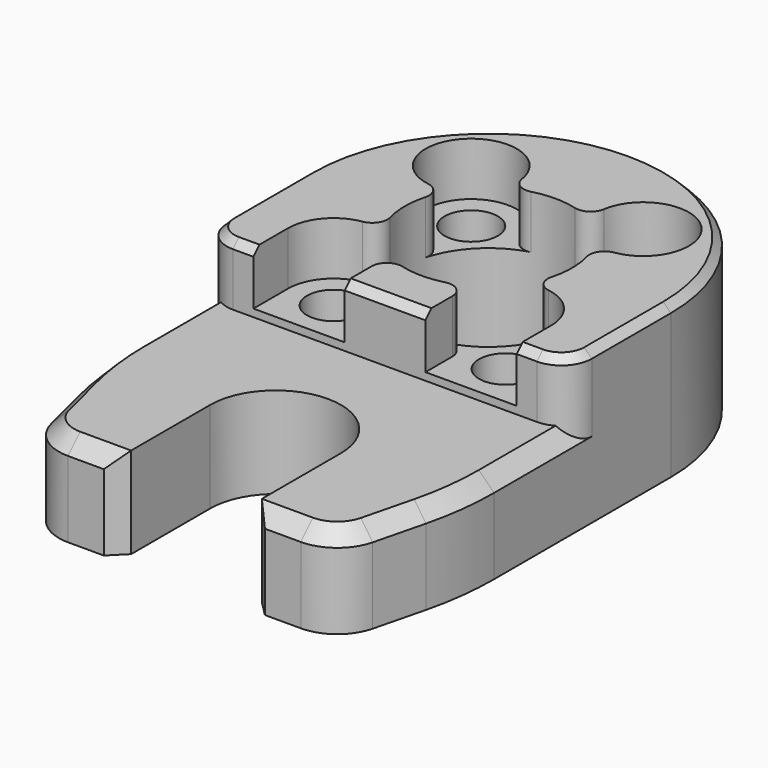
from build123d import *

# Parameters (mm, degrees)
F0_R        = 1.75
F0_R_2      = 5.5
F1_DEPTH    = 10
F2_SIZE2    = 8
F2_SIZE     = 2
F3_SIZE2    = 2
F3_SIZE     = 8
F5_W        = 20
F5_H        = 8
F6_DEPTH    = 15
F7_R        = 3
F8_DEPTH    = 3.5
F9_T1_DEPTH = 7.3998501729
F9_T3_DEPTH = 7.1931423334
F10_R       = 2
F11_SIZE    = 0.5
F12_SIZE    = 1
F13_R       = 3
F14_R       = 20
F15_SIZE    = 1
F17_ANGLE   = 45


# Not quite as in the source:
# - a fillet or chamfer that OpenCascade refuses, or shapes differently, is made with other operations: its cross-section is extruded or revolved along the edge and cut away or added


with BuildPart() as f1:
    # F0 (on Top) → F1 (new body)
    with BuildSketch(Plane.XY):
        with BuildLine():
            Line((-9.1923881554, -26.1629509039), (8.4852813742, -8.4852813742))
            ThreePointArc((8.4852813742, -8.4852813742), (8.4852813742, 8.4852813742), (-8.4852813742, 8.4852813742))
            Line((-8.4852813742, 8.4852813742), (-26.1629509039, -9.1923881554))
            Line((-26.1629509039, -9.1923881554), (-20.7182286888, -14.6371103706))
            Line((-20.7182286888, -14.6371103706), (-15.4149278299, -9.3338095117))
            ThreePointArc((-15.4149278299, -9.3338095117), (-9.3338095117, -9.3338095117), (-9.3338095117, -15.4149278299))
            Line((-9.3338095117, -15.4149278299), (-14.6371103706, -20.7182286888))
            Line((-14.6371103706, -20.7182286888), (-9.1923881554, -26.1629509039))
        make_face()
        with Locations((0, -8)):
            Circle(F0_R, mode=Mode.SUBTRACT)
        with Locations((-8, 0)):
            Circle(F0_R, mode=Mode.SUBTRACT)
        Circle(F0_R_2, mode=Mode.SUBTRACT)
        with Locations((8, 0)):
            Circle(F0_R, mode=Mode.SUBTRACT)
        with Locations((0, 8)):
            Circle(F0_R, mode=Mode.SUBTRACT)
    extrude(amount=F1_DEPTH)

    # F2
    f2_edges = [f1.edges().sort_by_distance(p)[0] for p in [
        (-26.162951, -9.192388, 5),
    ]]
    f2_side = f1.faces().sort_by_distance((-23.44059, -11.914749, 5))[0]
    chamfer(f2_edges, length=F2_SIZE, length2=F2_SIZE2, reference=f2_side)

    # F3
    f3_edges = [f1.edges().sort_by_distance(p)[0] for p in [
        (-9.192388, -26.162951, 5),
    ]]
    f3_side = f1.faces().sort_by_distance((-0.353553, -17.324116, 5))[0]
    chamfer(f3_edges, length=F3_SIZE, length2=F3_SIZE2, reference=f3_side)

    # F5 (on offset) → F6 (cut, symmetric)
    with BuildSketch(Plane(origin=(0.5303300859, -0.5303300859, 0), x_dir=(0.7071067812, 0.7071067812, 0), z_dir=(0.7071067812, -0.7071067812, 0))):
        with Locations((-18.5, 10)):
            Rectangle(F5_W, F5_H)
    extrude(amount=F6_DEPTH, both=True, mode=Mode.SUBTRACT)

    # F7 (on face) → F8 (cut)
    with BuildSketch(Plane.XY.offset(10)):
        with BuildLine():
            Line((-7.8890872965, -4.1317279836), (-5.8786796564, -2.1213203436))
            ThreePointArc((-5.8786796564, -2.1213203436), (-5.8786796564, 2.1213203436), (-10.1213203436, 2.1213203436))
            Line((-10.1213203436, 2.1213203436), (-12.1317279836, 0.1109127035))
            Line((-12.1317279836, 0.1109127035), (-7.8890872965, -4.1317279836))
        make_face()
        with BuildLine():
            Line((0.1109127035, -12.1317279836), (2.1213203436, -10.1213203436))
            ThreePointArc((2.1213203436, -10.1213203436), (2.1213203436, -5.8786796564), (-2.1213203436, -5.8786796564))
            Line((-2.1213203436, -5.8786796564), (-4.1317279836, -7.8890872965))
            Line((-4.1317279836, -7.8890872965), (0.1109127035, -12.1317279836))
        make_face()
        with Locations((8, 0)):
            Circle(F7_R)
        with Locations((0, 8)):
            Circle(F7_R)
    extrude(amount=-F8_DEPTH, mode=Mode.SUBTRACT)

    # F9: fillet of radius 1 on 8 edges, made by hand

    # F9_s2 → F9_t1 (cut)
    with BuildSketch(Plane.XY.offset(6.5)):
        with BuildLine():
            ThreePointArc((-6.3230487903, -2.5656894774), (-5.4874259536, -2.2810888302), (-4.7519509308, -2.7692891419))
            Line((-4.7519509308, -2.7692891419), (-4.665551823, -2.7189384302))
            ThreePointArc((-4.665551823, -2.7189384302), (-4.9962431034, -2.0487935111), (-5.23125, -1.3394116012))
            Line((-5.23125, -1.3394116012), (-5.4171875, -1.3187416691))
            ThreePointArc((-5.4171875, -1.3187416691), (-5.9493903346, -2.0506096654), (-6.3937594684, -2.4949787993))
            Line((-6.3937594684, -2.4949787993), (-6.3230487903, -2.5656894774))
        make_face()
        with BuildLine():
            ThreePointArc((-2.5656894774, -6.3230487903), (-2.2810888302, -5.4874259536), (-2.7692891419, -4.7519509308))
            Line((-2.7692891419, -4.7519509308), (-2.7189384302, -4.665551823))
            ThreePointArc((-2.7189384302, -4.665551823), (-2.0487935111, -4.9962431034), (-1.3394116012, -5.23125))
            Line((-1.3394116012, -5.23125), (-1.3187416691, -5.4171875))
            ThreePointArc((-1.3187416691, -5.4171875), (-2.0506096654, -5.9493903346), (-2.4949787993, -6.3937594684))
            Line((-2.4949787993, -6.3937594684), (-2.5656894774, -6.3230487903))
        make_face()
    extrude(amount=F9_T1_DEPTH, mode=Mode.SUBTRACT)

    # F9_s4 → F9_t3 (cut)
    with BuildSketch(Plane.XY.offset(6.5)):
        with BuildLine():
            ThreePointArc((-6.23046875, 2.4225521987), (-5.4322290759, 2.2520250497), (-4.7728365385, 2.7331358139))
            ThreePointArc((-4.7728365385, 2.7331358139), (-5.0966500462, 2.06740376), (-5.328125, 1.3642155198))
            ThreePointArc((-5.328125, 1.3642155198), (-5.717119911, 1.9463962852), (-6.23046875, 2.4225521987))
        make_face()
        with BuildLine():
            ThreePointArc((2.4225521987, -6.23046875), (2.2520250497, -5.4322290759), (2.7331358139, -4.7728365385))
            ThreePointArc((2.7331358139, -4.7728365385), (2.06740376, -5.0966500462), (1.3642155198, -5.328125))
            ThreePointArc((1.3642155198, -5.328125), (1.9463962852, -5.717119911), (2.4225521987, -6.23046875))
        make_face()
        with BuildLine():
            ThreePointArc((6.23046875, -2.4225521987), (5.4322290759, -2.2520250497), (4.7728365385, -2.7331358139))
            ThreePointArc((4.7728365385, -2.7331358139), (5.0966500462, -2.06740376), (5.328125, -1.3642155198))
            ThreePointArc((5.328125, -1.3642155198), (5.717119911, -1.9463962852), (6.23046875, -2.4225521987))
        make_face()
        with BuildLine():
            ThreePointArc((6.23046875, 2.4225521987), (5.4322290759, 2.2520250497), (4.7728365385, 2.7331358139))
            ThreePointArc((4.7728365385, 2.7331358139), (5.0966500462, 2.06740376), (5.328125, 1.3642155198))
            ThreePointArc((5.328125, 1.3642155198), (5.717119911, 1.9463962852), (6.23046875, 2.4225521987))
        make_face()
        with BuildLine():
            ThreePointArc((-2.4225521987, 6.23046875), (-2.2520250497, 5.4322290759), (-2.7331358139, 4.7728365385))
            ThreePointArc((-2.7331358139, 4.7728365385), (-2.06740376, 5.0966500462), (-1.3642155198, 5.328125))
            ThreePointArc((-1.3642155198, 5.328125), (-1.9463962852, 5.717119911), (-2.4225521987, 6.23046875))
        make_face()
        with BuildLine():
            ThreePointArc((2.4225521987, 6.23046875), (2.2520250497, 5.4322290759), (2.7331358139, 4.7728365385))
            ThreePointArc((2.7331358139, 4.7728365385), (2.06740376, 5.0966500462), (1.3642155198, 5.328125))
            ThreePointArc((1.3642155198, 5.328125), (1.9463962852, 5.717119911), (2.4225521987, 6.23046875))
        make_face()
    extrude(amount=F9_T3_DEPTH, mode=Mode.SUBTRACT)

    # F10
    f10_edges = [f1.edges().sort_by_distance(p)[0] for p in [
        (2.474874, -14.495689, 8),
        (-14.495689, 2.474874, 8),
    ]]
    fillet(f10_edges, radius=F10_R)

    # F11
    f11_edges = [f1.edges().sort_by_distance(p)[0] for p in [
        (0.585786, -12.606602, 10),
        (-12.606602, 0.585786, 10),
        (-6.010408, -6.010408, 10),
        (2.474874, -13.667262, 10),
        (-13.667262, 2.474874, 10),
        (6.187184, -10.783378, 10),
        (8.485281, 8.485281, 10),
        (-10.783378, 6.187184, 10),
    ]]
    chamfer(f11_edges, length=F11_SIZE)

    # F12
    f12_edges = [f1.edges().sort_by_distance(p)[0] for p in [
        (-20.718229, -14.63711, 3),
        (-14.63711, -20.718229, 3),
    ]]
    chamfer(f12_edges, length=F12_SIZE)

    # F13
    f13_edges = [f1.edges().sort_by_distance(p)[0] for p in [
        (-10.606602, -24.748737, 3),
        (-24.748737, -10.606602, 3),
    ]]
    fillet(f13_edges, radius=F13_R)

    # F14
    f14_edges = [f1.edges().sort_by_distance(p)[0] for p in [
        (-3.535534, -20.506097, 3),
        (-20.506097, -3.535534, 3),
    ]]
    fillet(f14_edges, radius=F14_R)

    # F15
    f15_edges = [f1.edges().sort_by_distance(p)[0] for p in [
        (-13.096441, -22.258898, 6),
        (-10.508108, -23.948663, 6),
        (-7.122424, -22.658231, 6),
        (-3.628449, -20.387093, 6),
        (0.340158, -16.630405, 6),
        (-22.258898, -13.096441, 6),
        (-23.948663, -10.508108, 6),
        (-22.658231, -7.122424, 6),
    ]]
    chamfer(f15_edges, length=F15_SIZE)


with BuildPart() as f1_1:
    # F17: moved
    add(f1.part.rotate(Axis((0, 0, 12.5), (0, 0, 1)), F17_ANGLE))


solid = f1_1.part
